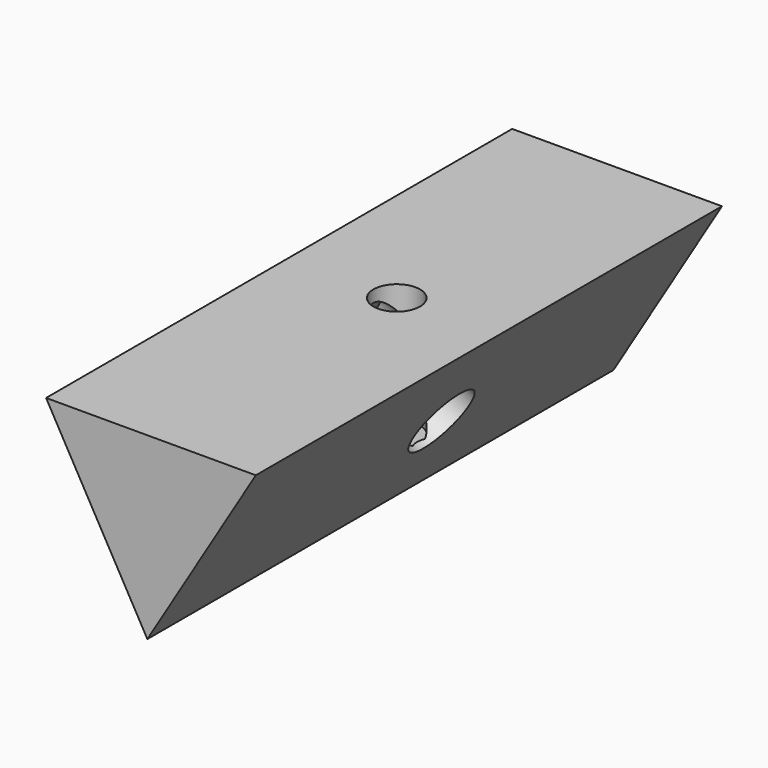
from build123d import *

# Parameters (mm, degrees)
F1_DEPTH = 50
F2_R     = 3
F5_DEPTH = 9.24953
F3_R     = 2
F6_DEPTH = 10.30413
F4_R     = 1.5
F7_DEPTH = 9.13494


with BuildPart() as f1:
    # F0 (on Front) → F1 (new body)
    with BuildSketch(Plane.XZ):
        Polygon((-9.2966205801, 5.7323870165), (-0.6050675001, -9.6636938179), (8.7033765413, 5.7425669072), align=None)
    extrude(amount=F1_DEPTH)

    # F2 (on face) → F5 (cut)
    with BuildSketch(Plane(origin=(3.8340726786, 0, -2.3165420615), x_dir=(0, 1, 0), z_dir=(0.8559033736, 0, -0.5171357801))):
        with Locations((-24, 0)):
            Circle(F2_R)
    extrude(amount=-F5_DEPTH, mode=Mode.SUBTRACT)

    # F3 (on face) → F6 (cut)
    with BuildSketch(Plane(origin=(-0.0032449215, 0, 5.7376428811), x_dir=(0.9999998401, 0, 0.0005655495), z_dir=(-0.0005655495, 0, 0.9999998401))):
        with Locations((0, -24)):
            Circle(F3_R)
    extrude(amount=-F6_DEPTH, mode=Mode.SUBTRACT)

    # F4 (on face) → F7 (cut)
    with BuildSketch(Plane(origin=(-4.5958448678, 0, -2.5944933678), x_dir=(0, -1, 0), z_dir=(-0.8708190517, 0, -0.491603681))):
        with Locations((24, 0)):
            Circle(F4_R)
    extrude(amount=-F7_DEPTH, mode=Mode.SUBTRACT)


solid = f1.part
